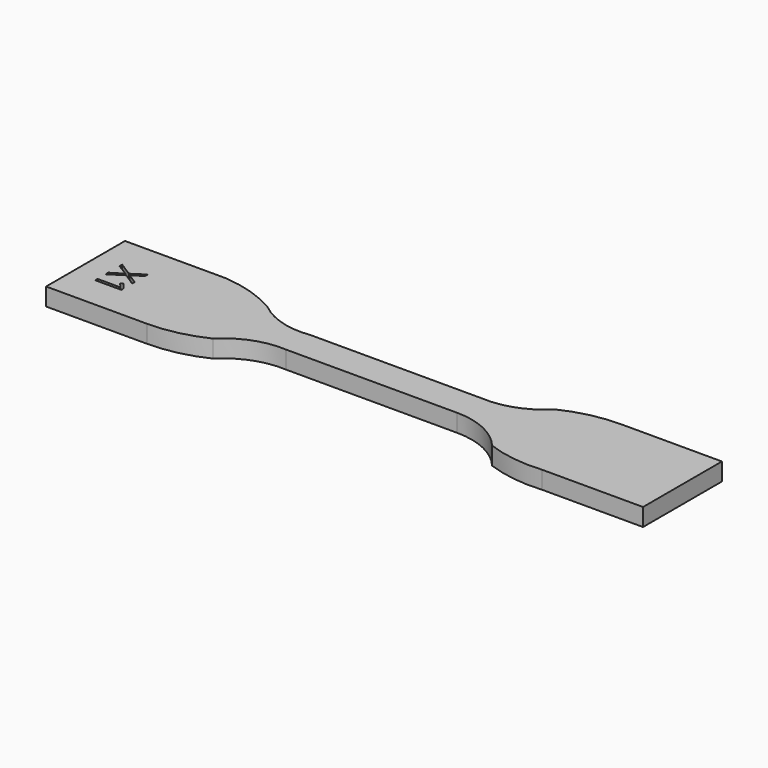
from build123d import *

# Parameters (mm, degrees)
F1_DEPTH     = 3.4
F2_TEXT_SIZE = 7.0564552314
F3_DEPTH     = 1


# Not quite as in the source:
# - Text() gives the source's letters only with a copy of the font that has no kerning and outlines rounded to 1/6400 em; it was checked with that copy


with BuildPart() as f1:
    # F0 (on Top) → F1 (new body)
    with BuildSketch(Plane.XY):
        with BuildLine():
            Line((-14.4320548165, 19.7811394548), (-33.8720548165, 19.7811394548))
            Line((-33.8720548165, 19.7811394548), (-33.8720548165, 0.7811394548))
            Line((-33.8720548165, 0.7811394548), (-14.4320548165, 0.7811394548))
            ThreePointArc((-14.4320548165, 0.7811394548), (-8.9053122052, 1.3996892086), (-3.6520548165, 3.2247301661))
            ThreePointArc((-3.6520548165, 3.2247301661), (1.3014698263, 6.4128780055), (7.1279451835, 7.2811394548))
            Line((7.1279451835, 7.2811394548), (40.1279451835, 7.2811394548))
            ThreePointArc((40.1279451835, 7.2811394548), (46.0837574042, 5.9511158081), (50.9079451835, 2.2137538538))
            ThreePointArc((50.9079451835, 2.2137538538), (56.2191047011, 0.9041953221), (61.6879451835, 0.7811394548))
            Line((61.6879451835, 0.7811394548), (81.1279451835, 0.7811394548))
            Line((81.1279451835, 0.7811394548), (81.1279451835, 19.7811394548))
            Line((81.1279451835, 19.7811394548), (61.6879451835, 19.7811394548))
            ThreePointArc((61.6879451835, 19.7811394548), (56.1612025723, 19.162589701), (50.9079451835, 17.3375487435))
            ThreePointArc((50.9079451835, 17.3375487435), (45.9544205407, 14.1494009041), (40.1279451835, 13.2811394548))
            Line((40.1279451835, 13.2811394548), (7.1279451835, 13.2811394548))
            ThreePointArc((7.1279451835, 13.2811394548), (1.4167452884, 13.6925537245), (-3.6520548165, 16.3560723447))
            ThreePointArc((-3.6520548165, 16.3560723447), (-8.8458057958, 18.686276846), (-14.4320548165, 19.7811394548))
        make_face()
    extrude(amount=F1_DEPTH)

    # F2 (on face) → F3 (cut)
    with BuildSketch(Plane.XY.offset(3.4)):
        with Locations(Location((-29.3886531144, 13.5272191837), (0, 0, -90))):
            Text('X1', F2_TEXT_SIZE, font='Open Sans', text_align=(TextAlign.LEFT, TextAlign.BOTTOM))
    extrude(amount=-F3_DEPTH, mode=Mode.SUBTRACT)


solid = f1.part
